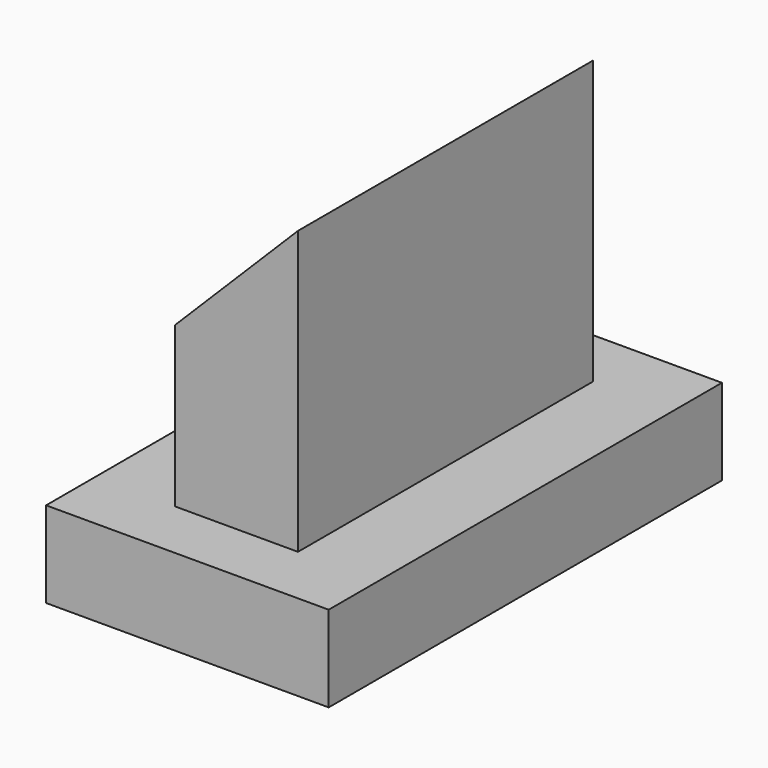
from build123d import *

# Parameters (mm, degrees)
F0_W     = 23
F0_H     = 40
F1_DEPTH = 7
F2_W     = 10
F2_H     = 30
F3_DEPTH = 30
F5_DEPTH = 0.4
F6_SIZE  = 9.99999


# Not quite as in the source:
# - a fillet or chamfer is up to 0.001 mm smaller than in the source, because OpenCascade refuses the exact size


with BuildPart() as f1:
    # F0 (on Top) → F1 (new body)
    with BuildSketch(Plane.XY):
        with Locations((11.5, 20)):
            Rectangle(F0_W, F0_H)
    extrude(amount=F1_DEPTH)

    # F2 (on Top) → F3 (join)
    with BuildSketch(Plane.XY):
        with Locations((11.5, 20)):
            Rectangle(F2_W, F2_H)
    extrude(amount=F3_DEPTH)

    # F4 (on Top) → F5 (cut)
    with BuildSketch(Plane.XY):
        Polygon((8, 17.75), (8, 2), (15, 2), (15, 17.75), (21, 17.75), (21, 22.25), (15, 22.25), (15, 37), (8, 37), (8, 22.25), (2, 22.25), (2, 17.75), align=None)
    extrude(amount=F5_DEPTH, mode=Mode.SUBTRACT)

    # F6 (size 10 in the source; OpenCascade refuses exactly that, so slightly less here)
    f6_edges = [f1.edges().sort_by_distance(p)[0] for p in [
        (6.5, 20, 30),
    ]]
    chamfer(f6_edges, length=F6_SIZE)


solid = f1.part
